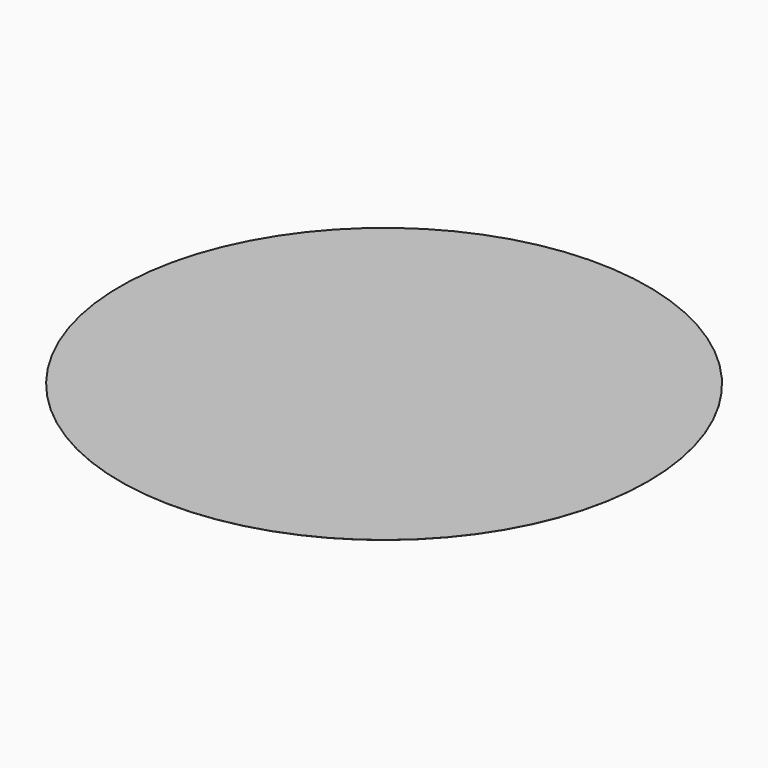
from build123d import *

# Parameters (mm, degrees)
F0_R     = 3048
F1_DEPTH = 0.79375


# Not quite as in the source:
# - a length typed as a fraction of an inch, garbled in the dataset ("3 / 203.2 mm" for 3/8 in), is restored


with BuildPart() as f1:
    # F0 (on Top) → F1 (new body)
    with BuildSketch(Plane.XY):
        Circle(F0_R)
    extrude(amount=F1_DEPTH)


solid = f1.part
